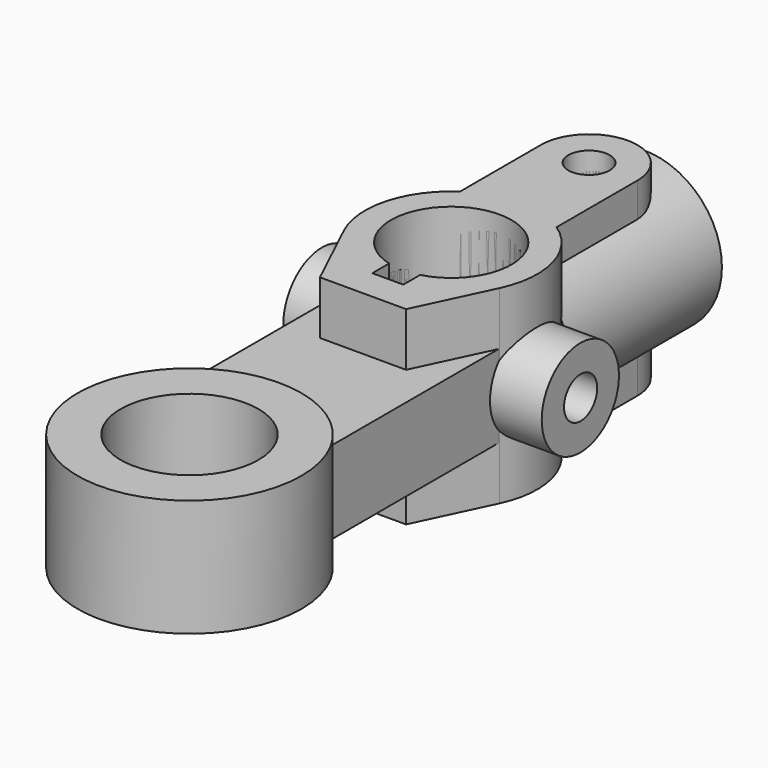
from build123d import *

# Parameters (mm, degrees)
F0_R      = 32.5
F0_R_2    = 20
F1_DEPTH  = 17
F4_DEPTH  = 22.5
F5_R      = 20
F6_DEPTH  = 50
F8_R      = 14
F9_DEPTH  = 75
F10_R     = 6.0012278007
F11_DEPTH = 75.001
F13_R     = 22.5
F14_DEPTH = 56
F15_R     = 11.5
F16_DEPTH = 56
F19_DEPTH = 55
F20_R     = 6
F21_DEPTH = 55.001
F22_R     = 6.0134317749
F23_DEPTH = 75.0010001


with BuildPart() as f1:
    # F0 (on Top) → F1 (new body, symmetric)
    with BuildSketch(Plane.XY):
        Circle(F0_R)
        Circle(F0_R_2, mode=Mode.SUBTRACT)
    extrude(amount=F1_DEPTH, both=True)

    # F3 (on Right) → F4 (join, symmetric)
    with BuildSketch(Plane.YZ):
        Polygon((0, 12), (0, 0), (0, -12), (95, -12), (95, 12), align=None)
    extrude(amount=F4_DEPTH, both=True)

    # F5 (on face) → F6 (cut, symmetric)
    with BuildSketch(Plane.XY):
        Circle(F5_R)
    extrude(amount=F6_DEPTH, both=True, mode=Mode.SUBTRACT)


with BuildPart() as f9:
    # F8 (on offset) → F9 (new body)
    with BuildSketch(Plane(origin=(-37.5, 0, 0), x_dir=(0, -1, 0), z_dir=(-1, 0, 0))):
        with Locations((-94.8872938752, 0)):
            Circle(F8_R)
    extrude(amount=-F9_DEPTH)


with BuildPart() as f11_tool:
    # F10 (on offset) → F11 (new body, through all)
    with BuildSketch(Plane(origin=(-37.5, 0, 0), x_dir=(0, -1, 0), z_dir=(-1, 0, 0))):
        with Locations((-94.9942693114, 0)):
            Circle(F10_R)
    extrude(amount=-F11_DEPTH)


with BuildPart() as f1_1:
    add(f1.part)

    # F11: cut by f11_tool
    add(f11_tool.part, mode=Mode.SUBTRACT)


with BuildPart() as f9_1:
    add(f9.part)

    # F11: cut by f11_tool
    add(f11_tool.part, mode=Mode.SUBTRACT)


with BuildPart() as f14:
    # F13 (on offset) → F14 (new body)
    with BuildSketch(Plane.XZ.offset(-165)):
        Circle(F13_R)
    extrude(amount=F14_DEPTH)

    # F15 (on offset) → F16 (cut)
    with BuildSketch(Plane.XZ.offset(-165)):
        Circle(F15_R)
    extrude(amount=F16_DEPTH, mode=Mode.SUBTRACT)


with BuildPart() as f19:
    # F18 (on offset) → F19 (new body)
    with BuildSketch(Plane.XY.offset(27.5)):
        with BuildLine():
            Line((12.5, 62.9366189241), (22.59139561, 84.2301328343))
            ThreePointArc((22.59139561, 84.2301328343), (24.1146807243, 101.5307203461), (14, 115.6489341013))
            Line((14, 115.6489341013), (14, 144.9366189241))
            ThreePointArc((14, 144.9366189241), (0, 158.9366189241), (-14, 144.9366189241))
            Line((-14, 144.9366189241), (-14, 115.6489341013))
            ThreePointArc((-14, 115.6489341013), (-24.1146807243, 101.5307203461), (-22.59139561, 84.2301328343))
            Line((-22.59139561, 84.2301328343), (-12.5, 62.9366189241))
            Line((-12.5, 62.9366189241), (0, 62.9366189241))
            Line((0, 62.9366189241), (12.5, 62.9366189241))
        make_face()
    extrude(amount=-F19_DEPTH)


with BuildPart() as f21_tool:
    # F20 (on face) → F21 (new body, through all)
    with BuildSketch(Plane.XY.offset(27.5)):
        with Locations((0, 144.9366189241)):
            Circle(F20_R)
        with BuildLine():
            Line((4.5, 71.9366189241), (4.5, 78.0250843989))
            ThreePointArc((4.5, 78.0250843989), (0, 112.4366189241), (-4.5, 78.0250843989))
            Line((-4.5, 78.0250843989), (-4.5, 71.9366189241))
            Line((-4.5, 71.9366189241), (0, 71.9366189241))
            Line((0, 71.9366189241), (4.5, 71.9366189241))
        make_face()
    extrude(amount=-F21_DEPTH)


with BuildPart() as f1_2:
    add(f1_1.part)

    # F21: cut by f21_tool
    add(f21_tool.part, mode=Mode.SUBTRACT)


with BuildPart() as f9_2:
    add(f9_1.part)

    # F21: cut by f21_tool
    add(f21_tool.part, mode=Mode.SUBTRACT)


with BuildPart() as f14_1:
    add(f14.part)

    # F21: cut by f21_tool
    add(f21_tool.part, mode=Mode.SUBTRACT)


with BuildPart() as f19_1:
    add(f19.part)

    # F21: cut by f21_tool
    add(f21_tool.part, mode=Mode.SUBTRACT)


with BuildPart() as f23_tool:
    # F22 (on offset) → F23 (new body, through all)
    with BuildSketch(Plane(origin=(-37.5, 0, 0), x_dir=(0, -1, 0), z_dir=(-1, 0, 0))):
        with Locations((-94.9962064624, 0)):
            Circle(F22_R)
    extrude(amount=-F23_DEPTH)


with BuildPart() as f1_3:
    add(f1_2.part)

    # F23: cut by f23_tool
    add(f23_tool.part, mode=Mode.SUBTRACT)


with BuildPart() as f9_3:
    add(f9_2.part)

    # F23: cut by f23_tool
    add(f23_tool.part, mode=Mode.SUBTRACT)


with BuildPart() as f19_2:
    add(f19_1.part)

    # F23: cut by f23_tool
    add(f23_tool.part, mode=Mode.SUBTRACT)


solid = Compound([f14_1.part, f1_3.part, f9_3.part, f19_2.part])
